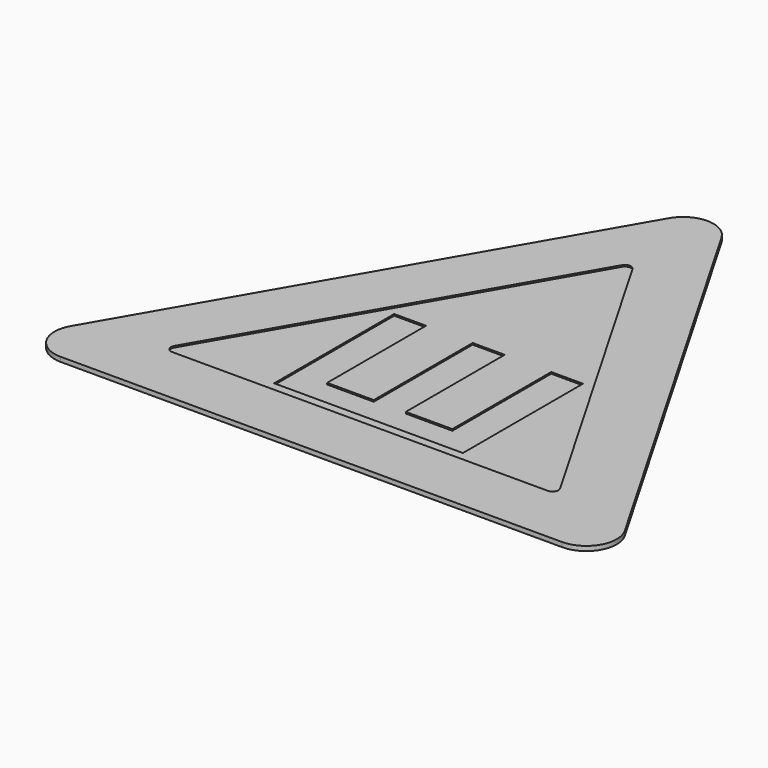
from build123d import *

# Parameters (mm, degrees)
F0_TEXT_SIZE = 69.3122098269
F1_DEPTH     = 0.5
F2_DEPTH     = 1
F3_DEPTH     = 1.5


# Not quite as in the source:
# - Text() gives the source's letters only with a copy of the font that has no kerning and outlines rounded to 1/6400 em; it was checked with that copy


with BuildPart() as f1:
    # F0 (on Top) → F1 (new body)
    with BuildSketch(Plane.XY):
        with BuildLine():
            Line((91.3397459622, -42.735026919), (8.6602540378, 100.4700538379))
            ThreePointArc((8.6602540378, 100.4700538379), (0, 105.4700538379), (-8.6602540378, 100.4700538379))
            Line((-8.6602540378, 100.4700538379), (-91.3397459622, -42.735026919))
            ThreePointArc((-91.3397459622, -42.735026919), (-91.3397459622, -52.735026919), (-82.6794919243, -57.735026919))
            Line((-82.6794919243, -57.735026919), (82.6794919243, -57.735026919))
            ThreePointArc((82.6794919243, -57.735026919), (91.3397459622, -52.735026919), (91.3397459622, -42.735026919))
        make_face()
        with BuildLine():
            ThreePointArc((-61.8948822335, -37.735026919), (-63.6269330411, -36.735026919), (-63.6269330411, -34.735026919))
            Line((-63.6269330411, -34.735026919), (-1.7320508076, 72.4700538379))
            ThreePointArc((-1.7320508076, 72.4700538379), (0, 73.4700538379), (1.7320508076, 72.4700538379))
            Line((1.7320508076, 72.4700538379), (63.6269330411, -34.735026919))
            ThreePointArc((63.6269330411, -34.735026919), (63.6269330411, -36.735026919), (61.8948822335, -37.735026919))
            Line((61.8948822335, -37.735026919), (-61.8948822335, -37.735026919))
        make_face(mode=Mode.SUBTRACT)
        with BuildLine():
            Line((-1.7320508076, 72.4700538379), (-63.6269330411, -34.735026919))
            ThreePointArc((-63.6269330411, -34.735026919), (-63.6269330411, -36.735026919), (-61.8948822335, -37.735026919))
            Line((-61.8948822335, -37.735026919), (61.8948822335, -37.735026919))
            ThreePointArc((61.8948822335, -37.735026919), (63.6269330411, -36.735026919), (63.6269330411, -34.735026919))
            Line((63.6269330411, -34.735026919), (1.7320508076, 72.4700538379))
            ThreePointArc((1.7320508076, 72.4700538379), (0, 73.4700538379), (-1.7320508076, 72.4700538379))
        make_face()
        Polygon((5.3060179482, 15.2902489782), (5.3060179482, -25.4631643935), (20.663004438, -25.4631643935), (20.663004438, 15.2902489782), (31.1248161088, 15.2902489782), (31.1248161088, -34.1921708185), (-31.1153823092, -34.1921708185), (-31.1153823092, 15.2902489782), (-20.6210805401, 15.2902489782), (-20.6210805401, -25.4631643935), (-5.2532640176, -25.4631643935), (-5.2532640176, 15.2902489782), align=None, mode=Mode.SUBTRACT)
        with Locations((-37.3426511608, -34.1921708185)):
            Text('Ш', F0_TEXT_SIZE, font='Open Sans', font_style=FontStyle.BOLD, text_align=(TextAlign.LEFT, TextAlign.BOTTOM))
    extrude(amount=F1_DEPTH)


with BuildPart() as f2:
    # F0 (on Top) → F2 (new body)
    with BuildSketch(Plane.XY):
        with BuildLine():
            Line((91.3397459622, -42.735026919), (8.6602540378, 100.4700538379))
            ThreePointArc((8.6602540378, 100.4700538379), (0, 105.4700538379), (-8.6602540378, 100.4700538379))
            Line((-8.6602540378, 100.4700538379), (-91.3397459622, -42.735026919))
            ThreePointArc((-91.3397459622, -42.735026919), (-91.3397459622, -52.735026919), (-82.6794919243, -57.735026919))
            Line((-82.6794919243, -57.735026919), (82.6794919243, -57.735026919))
            ThreePointArc((82.6794919243, -57.735026919), (91.3397459622, -52.735026919), (91.3397459622, -42.735026919))
        make_face()
        with BuildLine():
            ThreePointArc((-61.8948822335, -37.735026919), (-63.6269330411, -36.735026919), (-63.6269330411, -34.735026919))
            Line((-63.6269330411, -34.735026919), (-1.7320508076, 72.4700538379))
            ThreePointArc((-1.7320508076, 72.4700538379), (0, 73.4700538379), (1.7320508076, 72.4700538379))
            Line((1.7320508076, 72.4700538379), (63.6269330411, -34.735026919))
            ThreePointArc((63.6269330411, -34.735026919), (63.6269330411, -36.735026919), (61.8948822335, -37.735026919))
            Line((61.8948822335, -37.735026919), (-61.8948822335, -37.735026919))
        make_face(mode=Mode.SUBTRACT)
        with BuildLine():
            Line((-1.7320508076, 72.4700538379), (-63.6269330411, -34.735026919))
            ThreePointArc((-63.6269330411, -34.735026919), (-63.6269330411, -36.735026919), (-61.8948822335, -37.735026919))
            Line((-61.8948822335, -37.735026919), (61.8948822335, -37.735026919))
            ThreePointArc((61.8948822335, -37.735026919), (63.6269330411, -36.735026919), (63.6269330411, -34.735026919))
            Line((63.6269330411, -34.735026919), (1.7320508076, 72.4700538379))
            ThreePointArc((1.7320508076, 72.4700538379), (0, 73.4700538379), (-1.7320508076, 72.4700538379))
        make_face()
        Polygon((5.3060179482, 15.2902489782), (5.3060179482, -25.4631643935), (20.663004438, -25.4631643935), (20.663004438, 15.2902489782), (31.1248161088, 15.2902489782), (31.1248161088, -34.1921708185), (-31.1153823092, -34.1921708185), (-31.1153823092, 15.2902489782), (-20.6210805401, 15.2902489782), (-20.6210805401, -25.4631643935), (-5.2532640176, -25.4631643935), (-5.2532640176, 15.2902489782), align=None, mode=Mode.SUBTRACT)
    extrude(amount=F2_DEPTH)


with BuildPart() as f3:
    # F0 (on Top) → F3 (new body)
    with BuildSketch(Plane.XY):
        with BuildLine():
            Line((91.3397459622, -42.735026919), (8.6602540378, 100.4700538379))
            ThreePointArc((8.6602540378, 100.4700538379), (0, 105.4700538379), (-8.6602540378, 100.4700538379))
            Line((-8.6602540378, 100.4700538379), (-91.3397459622, -42.735026919))
            ThreePointArc((-91.3397459622, -42.735026919), (-91.3397459622, -52.735026919), (-82.6794919243, -57.735026919))
            Line((-82.6794919243, -57.735026919), (82.6794919243, -57.735026919))
            ThreePointArc((82.6794919243, -57.735026919), (91.3397459622, -52.735026919), (91.3397459622, -42.735026919))
        make_face()
        with BuildLine():
            ThreePointArc((-61.8948822335, -37.735026919), (-63.6269330411, -36.735026919), (-63.6269330411, -34.735026919))
            Line((-63.6269330411, -34.735026919), (-1.7320508076, 72.4700538379))
            ThreePointArc((-1.7320508076, 72.4700538379), (0, 73.4700538379), (1.7320508076, 72.4700538379))
            Line((1.7320508076, 72.4700538379), (63.6269330411, -34.735026919))
            ThreePointArc((63.6269330411, -34.735026919), (63.6269330411, -36.735026919), (61.8948822335, -37.735026919))
            Line((61.8948822335, -37.735026919), (-61.8948822335, -37.735026919))
        make_face(mode=Mode.SUBTRACT)
    extrude(amount=F3_DEPTH)


solid = Compound([f1.part, f2.part, f3.part])
